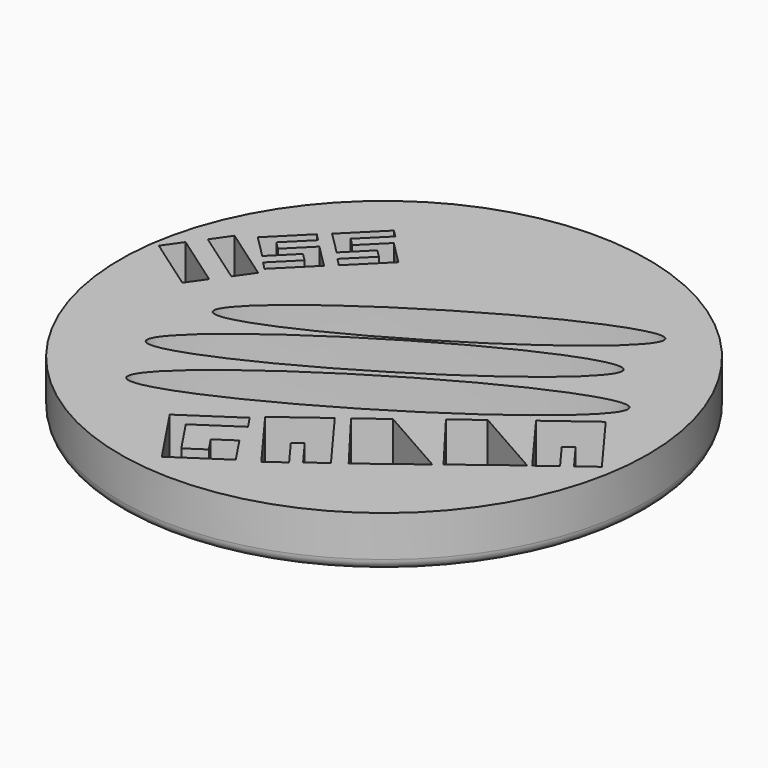
from build123d import *

# Parameters (mm, degrees)
F0_R     = 12.125
F2_DEPTH = 2.38


# Not quite as in the source:
# - a fillet or chamfer that OpenCascade refuses, or shapes differently, is made with other operations: its cross-section is extruded or revolved along the edge and cut away or added


with BuildPart() as f2:
    # F0 (on Top) → F2 (new body)
    with BuildSketch(Plane.XY):
        Circle(F0_R)
        Polygon((-3.2093067312, -8.296926559), (-0.8131807139, -6.6990929169), (-0.4216222868, -7.2856470722), (-2.2859056129, -8.5288265191), (-1.2460206689, -10.08824754), (-0.4216222869, -9.5385053896), (-0.8599218546, -8.8812273288), (0, -8.3077966916), (0.8322003947, -9.5557720532), (-1.3842535445, -11.0337930941), align=None, mode=Mode.SUBTRACT)
        Polygon((2.4562833268, -8.5223700524), (1.651227667, -9.1155693314), (-0.4249698094, -6.2978745219), (1.5810172705, -4.8058485212), (3.6572147468, -7.6235433307), (2.852159087, -8.2167426096), (1.9623601685, -7.0091591199), (1.5598323386, -7.3057587593), align=None, mode=Mode.SUBTRACT)
        Polygon((6.5659907646, -5.4407012337), (4.1779835818, -7.2565816525), (2.0594564267, -4.4705732726), (3.253460018, -3.5626330632), align=None, mode=Mode.SUBTRACT)
        with BuildLine():
            add(Edge.make_bspline(
                [(9.3386698082, 2.4187678684), (8.1497764129, 4.3790980975), (-2.9293388718, -3.6808031421), (-14.0084541566, -11.7407043817), (-1.7404454766, -5.6411333711), (10.5275632034, 0.4584376394), (9.3386698082, 2.4187678684)],
                knots=[0, 0, 0, 2.0943951024, 2.0943951024, 4.1887902048, 4.1887902048, 6.2831853072, 6.2831853072, 6.2831853072], degree=2, weights=[1, 0.5, 1, 0.5, 1, 0.5, 1]))
        make_face(mode=Mode.SUBTRACT)
        Polygon((9.2717871239, -3.3746159405), (6.8837799411, -5.1904963592), (4.7652527859, -2.4044879793), (5.9592563773, -1.49654777), align=None, mode=Mode.SUBTRACT)
        Polygon((10.230396352, -2.6835796259), (9.4253406921, -3.2767789049), (7.3491432158, -0.4590840954), (9.3551302956, 1.0329419053), (11.431327772, -1.7847529042), (10.6262721121, -2.3779521831), (9.7364731937, -1.1703686933), (9.3339453638, -1.4669683328), align=None, mode=Mode.SUBTRACT)
        Polygon((-9.252220741, -0.0182491862), (-11.7099159868, 1.7021385838), (-11.1364533968, 2.5213703323), (-8.678758151, 0.8009825624), align=None, mode=Mode.SUBTRACT)
        Polygon((-8.1887295845, 1.4652768326), (-10.6464248303, 3.1856646026), (-10.0729622403, 4.0048963511), (-7.6152669945, 2.2845085812), align=None, mode=Mode.SUBTRACT)
        Polygon((-9.347300169, 4.430499518), (-7.841588868, 5.936210455), (-7.5140006084, 5.6086221162), (-8.5829520327, 4.5396709503), (-8.2293986849, 4.186117517), (-7.1687383849, 5.2467775605), (-6.1080785977, 4.186117517), (-7.6266925716, 2.6671674091), (-7.9802459194, 3.0207208425), (-6.9195856195, 4.0813808861), (-7.2731389673, 4.4349343194), (-8.3124372196, 3.3956363184), align=None, mode=Mode.SUBTRACT)
        with BuildLine():
            add(Edge.make_bspline(
                [(7.3327392075, 4.5926569432), (6.2035325254, 6.4545715628), (-4.3193714297, -1.2006937226), (-14.8422753849, -8.855959008), (-3.1901647477, -3.0626083422), (8.4619458895, 2.7307423236), (7.3327392075, 4.5926569432)],
                knots=[0, 0, 0, 2.0943951024, 2.0943951024, 4.1887902048, 4.1887902048, 6.2831853072, 6.2831853072, 6.2831853072], degree=2, weights=[1, 0.5, 1, 0.5, 1, 0.5, 1]))
        make_face(mode=Mode.SUBTRACT)
        Polygon((-7.4380451802, 6.3134137932), (-5.8618537193, 7.8896048731), (-5.5342654597, 7.5620165344), (-6.6736970439, 6.4225852256), (-6.320143696, 6.0690317922), (-5.2594833961, 7.1296918358), (-4.1988236089, 6.0690317922), (-5.7174375827, 4.5500816844), (-6.0709909306, 4.9036351177), (-5.0103306306, 5.9642951613), (-5.3638839785, 6.3178485947), (-6.4031822307, 5.2785505936), align=None, mode=Mode.SUBTRACT)
        with BuildLine():
            add(Edge.make_bspline(
                [(7.0022831521, 7.3981736055), (5.9325623329, 9.1620037916), (-4.0360019856, 1.9100128299), (-14.0045663042, -5.3419781317), (-2.9662811665, 0.1461826439), (8.0720039713, 5.6343434195), (7.0022831521, 7.3981736055)],
                knots=[0, 0, 0, 2.0943951024, 2.0943951024, 4.1887902048, 4.1887902048, 6.2831853072, 6.2831853072, 6.2831853072], degree=2, weights=[1, 0.5, 1, 0.5, 1, 0.5, 1]))
        make_face(mode=Mode.SUBTRACT)
    extrude(amount=F2_DEPTH)

    # F3: fillet of radius 0.5 on 1 edges, made by hand

    # F3_s1 → F3_t2 (revolve, cut)
    with BuildSketch(Plane.XZ):
        with BuildLine():
            ThreePointArc((12.125, 0.5), (11.9785533906, 0.1464466094), (11.625, 0))
            Line((11.625, 0), (12.125, 0))
            Line((12.125, 0), (12.125, 0.5))
        make_face()
    revolve(axis=Axis((0, 0, 0), (0, 0, 1)), mode=Mode.SUBTRACT)


solid = f2.part
